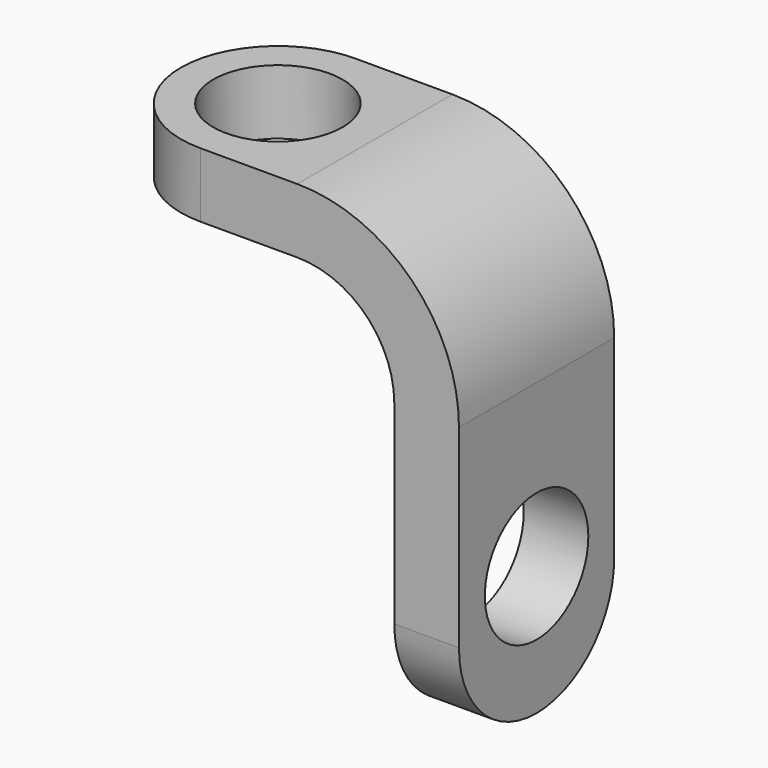
from build123d import *

# Parameters (mm, degrees)
F1_DEPTH = 7.5
F2_R     = 7.49999
F3_R     = 5
F4_DEPTH = 35.001
F5_R     = 5
F6_DEPTH = 27.501


# Not quite as in the source:
# - a fillet or chamfer is up to 0.001 mm smaller than in the source, because OpenCascade refuses the exact size


with BuildPart() as f1:
    # F0 (on Front) → F1 (new body, symmetric)
    with BuildSketch(Plane.XZ):
        with BuildLine():
            Line((7.5, 25), (-7.5, 25))
            Line((-7.5, 25), (-7.5, 20))
            Line((-7.5, 20), (7.5, 20))
            ThreePointArc((7.5, 20), (12.8033008589, 17.8033008589), (15, 12.5))
            Line((15, 12.5), (15, -10))
            Line((15, -10), (20, -10))
            Line((20, -10), (20, 12.5))
            ThreePointArc((20, 12.5), (16.3388347648, 21.3388347648), (7.5, 25))
        make_face()
    extrude(amount=F1_DEPTH, both=True)

    # F2 (radius 7.5 in the source; OpenCascade refuses exactly that, so slightly less here)
    f2_edges = [f1.edges().sort_by_distance(p)[0] for p in [
        (-7.5, -7.5, 22.5),
        (-7.5, 7.5, 22.5),
        (17.5, -7.5, -10),
        (17.5, 7.5, -10),
    ]]
    fillet(f2_edges, radius=F2_R)

    # F3 (on face) → F4 (cut, through all)
    with BuildSketch(Plane.XY.offset(25)):
        Circle(F3_R)
    extrude(amount=-F4_DEPTH, mode=Mode.SUBTRACT)

    # F5 (on face) → F6 (cut, through all)
    with BuildSketch(Plane.YZ.offset(20)):
        Circle(F5_R)
    extrude(amount=-F6_DEPTH, mode=Mode.SUBTRACT)


solid = f1.part
